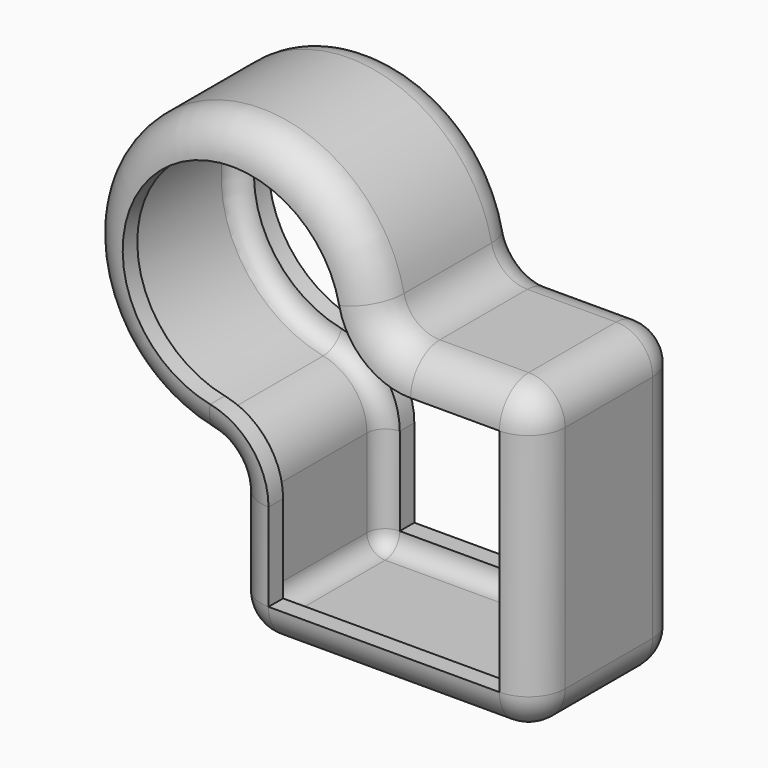
from build123d import *

# Parameters (mm, degrees)
F1_DEPTH = 25
F2_R     = 5
F3_T     = -2.5


# Not quite as in the source:
# - a shell that OpenCascade refuses in one call is made with other operations: the cavity is built on its own and cut out


with BuildPart() as f1:
    # F0 (on Front) → F1 (new body)
    with BuildSketch(Plane.XZ):
        with BuildLine():
            ThreePointArc((0, -20), (14.1421356237, -14.1421356237), (20, 0))
            Line((20, 0), (0, 0))
            Line((0, 0), (0, -20))
        make_face()
        with BuildLine():
            Line((41.6772402823, 0), (20, 0))
            ThreePointArc((20, 0), (14.1421356237, -14.1421356237), (0, -20))
            Line((0, -20), (0, -41.548602283))
            Line((0, -41.548602283), (41.6772402823, -41.548602283))
            Line((41.6772402823, -41.548602283), (41.6772402823, 0))
        make_face()
        with BuildLine():
            Line((0, 0), (20, 0))
            ThreePointArc((20, 0), (-14.1421356237, 14.1421356237), (0, -20))
            Line((0, -20), (0, 0))
        make_face()
    extrude(amount=F1_DEPTH)

    # F2
    f2_edges = [f1.edges().sort_by_distance(p)[0] for p in [
        (30.83862, -25, 0),
        (30.83862, 0, 0),
        (41.67724, -12.5, 0),
        (41.67724, -12.5, -41.548602),
        (41.67724, 0, -20.774301),
        (41.67724, -25, -20.774301),
        (0, 0, -30.774301),
        (0, -12.5, -41.548602),
        (20.83862, 0, -41.548602),
        (0, -25, -30.774301),
        (20.83862, -25, -41.548602),
        (-14.142136, -25, 14.142136),
        (20, -12.5, 0),
        (0, -12.5, -20),
        (-14.142136, 0, 14.142136),
    ]]
    fillet(f2_edges, radius=F2_R)

    # F3: a shell. OpenCascade refuses it in one call, so the cavity is built on its own and cut out:
    # the body offset inwards by the wall thickness, plus a prism from it out through each open face.
    f3_core = offset(f1.part, amount=F3_T, mode=Mode.PRIVATE)
    f3_exits = [f3_core.faces().sort_by_distance(p)[0] for p in [
        (12.277465, -22.5, -12.239423),
        (12.277465, -2.5, -12.239423),
    ]]
    add(f3_core, mode=Mode.SUBTRACT)
    extrude(f3_exits, amount=-F3_T, mode=Mode.SUBTRACT)


solid = f1.part
